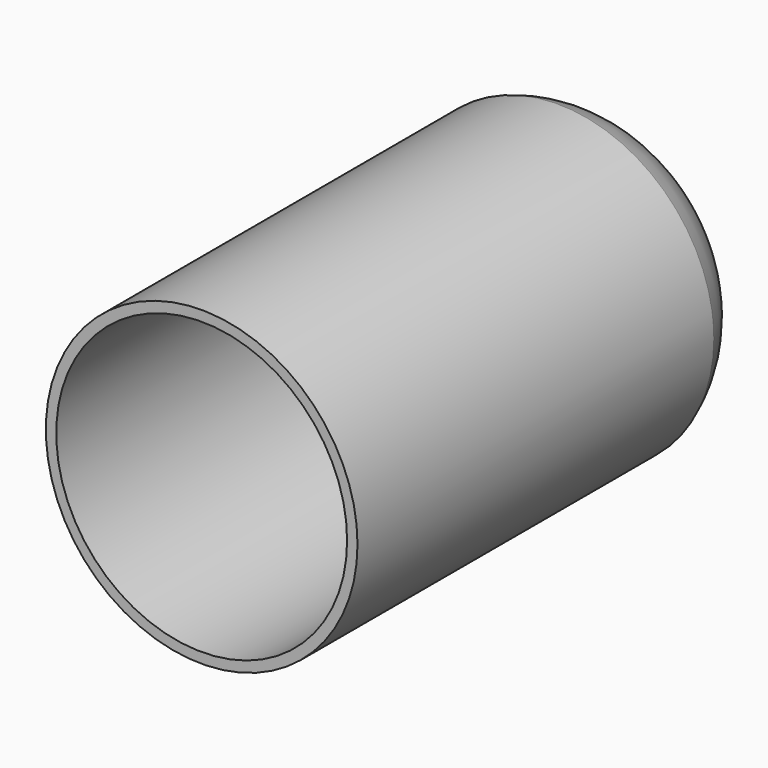
from build123d import *

# Parameters (mm, degrees)
F0_R     = 38.1
F1_DEPTH = 127
F6_T     = -2.54


# Not quite as in the source:
# - a feature of the source that left no trace in its solid (it failed there, or was rolled back) is left out


with BuildPart() as f1:
    # F0 (on Front) → F1 (new body)
    with BuildSketch(Plane.XZ):
        Circle(F0_R)
    extrude(amount=F1_DEPTH)

    # F2 (on Top) → F3 (revolve, cut)
    with BuildSketch(Plane.XY):
        with BuildLine():
            Line((-12.7, 0), (0, 0))
            Line((0, 0), (0, 26.976691559))
            Line((0, 26.976691559), (-68.359054625, 26.976691559))
            Line((-68.359054625, 26.976691559), (-68.359054625, -28.0306376517))
            Line((-68.359054625, -28.0306376517), (-39.5489111543, -28.0306376517))
            ThreePointArc((-39.5489111543, -28.0306376517), (-32.1073483334, -8.2846551837), (-12.7, 0))
        make_face()
    revolve(axis=Axis((0, 13.4883457795, 0), (0, -1, 0)), mode=Mode.SUBTRACT)

    # F6
    f6_openings = [f1.faces().sort_by_distance(p)[0] for p in [
        (0, -127, 0),
    ]]
    offset(amount=F6_T, openings=f6_openings)


solid = f1.part
